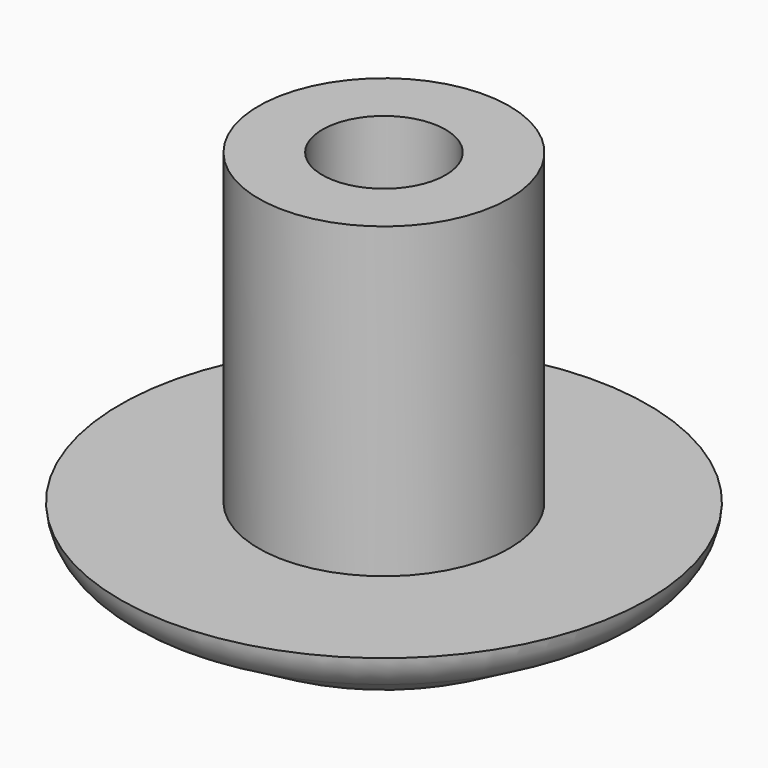
from build123d import *

# Parameters (mm, degrees)
F0_R     = 6
F1_DEPTH = 2
F2_SIZE2 = 2.5980762114
F2_SIZE  = 1.5
F4_R     = 2.85
F4_R_2   = 1.4
F5_DEPTH = 7
F6_R     = 1.2


# Not quite as in the source:
# - a fillet or chamfer that OpenCascade refuses, or shapes differently, is made with other operations: its cross-section is extruded or revolved along the edge and cut away or added


with BuildPart() as f1:
    # F0 (on Top) → F1 (new body)
    with BuildSketch(Plane.XY):
        Circle(F0_R)
    extrude(amount=F1_DEPTH)

    # F2
    f2_edges = [f1.edges().sort_by_distance(p)[0] for p in [
        (-6, 0, 0),
    ]]
    f2_side = f1.faces().sort_by_distance((-6, 0, 1))[0]
    chamfer(f2_edges, length=F2_SIZE, length2=F2_SIZE2, reference=f2_side)

    # F3: fillet of radius 1 on 2 edges, made by hand

    # F3_s1 → F3_t2 (revolve, cut)
    with BuildSketch(Plane.XZ):
        with BuildLine():
            ThreePointArc((3.6339745962, 0.1339745962), (3.3927936413, 0.0340741737), (3.1339745962, 0))
            Line((3.1339745962, 0), (3.4019237886, 0))
            Line((3.4019237886, 0), (3.6339745962, 0.1339745962))
        make_face()
    revolve(axis=Axis((0, 0, 0), (0, 0, 1)), mode=Mode.SUBTRACT)

    # F3_s3 → F3_t4 (revolve, cut)
    with BuildSketch(Plane.XZ):
        with BuildLine():
            ThreePointArc((6, 2), (5.8486778537, 1.5452494356), (5.5031382462, 1.2131367327))
            Line((5.5031382462, 1.2131367327), (6, 1.5))
            Line((6, 1.5), (6, 2))
        make_face()
    revolve(axis=Axis((0, 0, 1.5), (0, 0, 1)), mode=Mode.SUBTRACT)

    # F4 (on face) → F5 (join)
    with BuildSketch(Plane.XY.offset(2)):
        Circle(F4_R)
        Circle(F4_R_2, mode=Mode.SUBTRACT)
    extrude(amount=F5_DEPTH)

    # F6
    f6_edges = [f1.edges().sort_by_distance(p)[0] for p in [
        (-1.4, 0, 2),
    ]]
    fillet(f6_edges, radius=F6_R)


solid = f1.part
